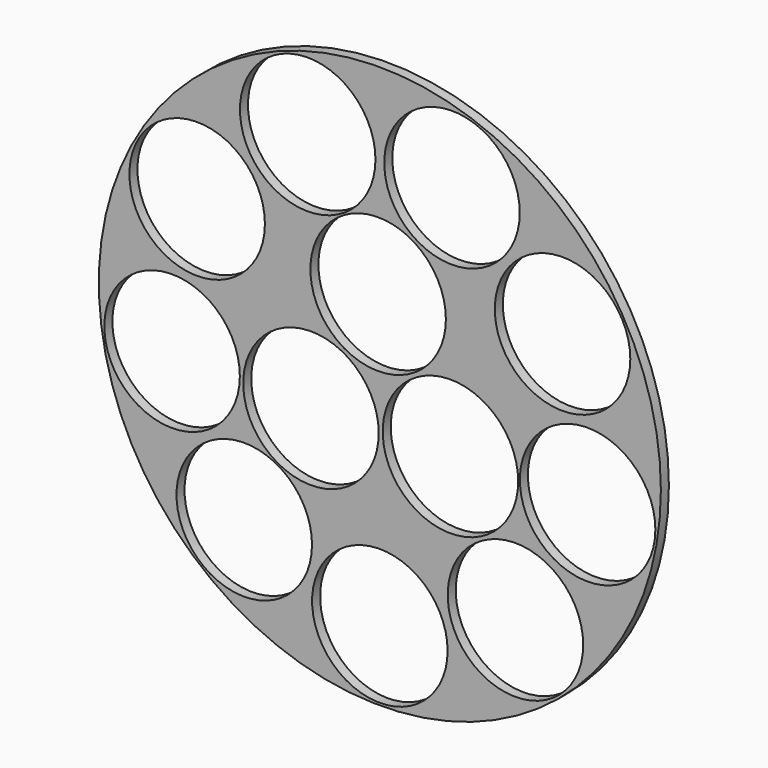
from build123d import *

# Parameters (mm, degrees)
F0_R     = 84
F0_R_2   = 20.25
F1_DEPTH = 3


# Not quite as in the source:
# - a feature of the source that left no trace in its solid (it failed there, or was rolled back) is left out


with BuildPart() as f1:
    # F0 (on Front) → F1 (new body)
    with BuildSketch(Plane.XZ):
        with Locations((188.1058226409, 180.2671665321)):
            Circle(F0_R)
        with Locations((147.5744029219, 131.9637014691)):
            Circle(F0_R_2, mode=Mode.SUBTRACT)
        with Locations((126.008084946, 169.3176599356)):
            Circle(F0_R_2, mode=Mode.SUBTRACT)
        with Locations((188.1058226409, 117.2114711388)):
            Circle(F0_R_2, mode=Mode.SUBTRACT)
        with Locations((228.6372423598, 131.9637014691)):
            Circle(F0_R_2, mode=Mode.SUBTRACT)
        with Locations((167.5180891549, 167.7861717837)):
            Circle(F0_R_2, mode=Mode.SUBTRACT)
        with Locations((209.2085479005, 168.6781637011)):
            Circle(F0_R_2, mode=Mode.SUBTRACT)
        with Locations((250.2035603357, 169.3176599356)):
            Circle(F0_R_2, mode=Mode.SUBTRACT)
        with Locations((133.497988577, 211.7950142288)):
            Circle(F0_R_2, mode=Mode.SUBTRACT)
        with Locations((187.5908308672, 204.3371641115)):
            Circle(F0_R_2, mode=Mode.SUBTRACT)
        with Locations((242.7136567047, 211.7950142288)):
            Circle(F0_R_2, mode=Mode.SUBTRACT)
        with Locations((166.539504665, 239.5201381917)):
            Circle(F0_R_2, mode=Mode.SUBTRACT)
        with Locations((209.6721406168, 239.5201381917)):
            Circle(F0_R_2, mode=Mode.SUBTRACT)
    extrude(amount=F1_DEPTH)


solid = f1.part
